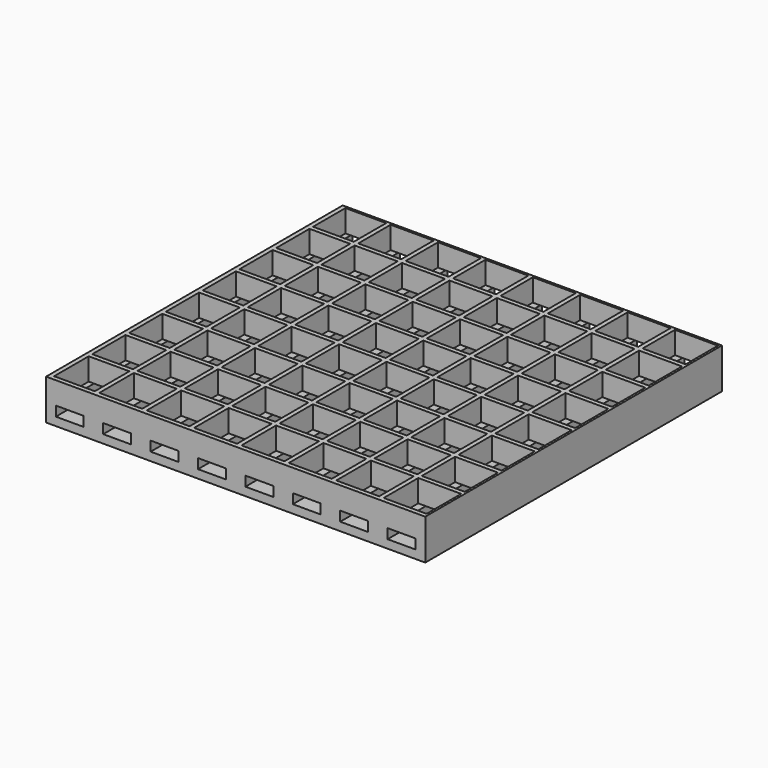
from build123d import *

# Parameters (mm, degrees)
F0_W                 = 3.5
F0_H                 = 3.5
F0_W_2               = 7
F1_DEPTH             = 133
F2_W                 = 1.6
F2_H                 = 8
F2_W_2               = 0.8
F3_DEPTH             = 133
F4_W                 = 0.8
F4_H                 = 8
F4_W_2               = 1.6
F5_DEPTH             = 136
F8_D                 = 3.5
F8_DEPTH             = 12
F8_CSINK_D           = 6.5
F8_CSINK_ANGLE       = 90
F8_TIP               = 1.0515060833
F8_ON_F6_D           = 3.5
F8_ON_F6_DEPTH       = 12
F8_ON_F6_CSINK_D     = 6.5
F8_ON_F6_CSINK_ANGLE = 90
F8_ON_F6_TIP         = 1.0515060833


# Not quite as in the source:
# - a feature names something its author has since deleted; it is built from what else it names


with BuildPart() as f1:
    # F0 (on Front) → F1 (new body)
    with BuildSketch(Plane.XZ):
        with Locations((-66.25, 4.75)):
            Rectangle(F0_W, F0_H)
        with Locations((-17, 4.75)):
            Rectangle(F0_W_2, F0_H)
        with Locations((66.25, 4.75)):
            Rectangle(F0_W, F0_H)
        Polygon((-64.5, 3), (-68, 3), (-68, 0), (68, 0), (68, 3), (64.5, 3), (54.5, 3), (47.5, 3), (37.5, 3), (30.5, 3), (20.5, 3), (13.5, 3), (3.5, 3), (-3.5, 3), (-13.5, 3), (-20.5, 3), (-30.5, 3), (-37.5, 3), (-47.5, 3), (-54.5, 3), align=None)
        with Locations((-51, 4.75)):
            Rectangle(F0_W_2, F0_H)
        with Locations((-34, 4.75)):
            Rectangle(F0_W_2, F0_H)
        with Locations((0, 4.75)):
            Rectangle(F0_W_2, F0_H)
        with Locations((17, 4.75)):
            Rectangle(F0_W_2, F0_H)
        with Locations((34, 4.75)):
            Rectangle(F0_W_2, F0_H)
        with Locations((51, 4.75)):
            Rectangle(F0_W_2, F0_H)
    extrude(amount=F1_DEPTH)

    # F2 (on face) → F3 (join, through all)
    with BuildSketch(Plane.XZ.offset(133)):
        with Locations((-67.2, 10.5)):
            Rectangle(F2_W, F2_H)
        with Locations((-51, 10.5)):
            Rectangle(F2_W, F2_H)
        with Locations((-34, 10.5)):
            Rectangle(F2_W, F2_H)
        with Locations((-17, 10.5)):
            Rectangle(F2_W, F2_H)
        with Locations((0, 10.5)):
            Rectangle(F2_W, F2_H)
        with Locations((17, 10.5)):
            Rectangle(F2_W, F2_H)
        with Locations((34, 10.5)):
            Rectangle(F2_W, F2_H)
        with Locations((51, 10.5)):
            Rectangle(F2_W, F2_H)
        with Locations((67.6, 10.5)):
            Rectangle(F2_W_2, F2_H)
    extrude(amount=-F3_DEPTH)

    # F4 (on face) → F5 (join, through all)
    with BuildSketch(Plane(origin=(-68, 0, 0), x_dir=(0, -1, 0), z_dir=(-1, 0, 0))):
        with Locations((0.4, 10.5)):
            Rectangle(F4_W, F4_H)
        with Locations((16.1, 10.5)):
            Rectangle(F4_W_2, F4_H)
        with Locations((32.6, 10.5)):
            Rectangle(F4_W_2, F4_H)
        with Locations((49.1, 10.5)):
            Rectangle(F4_W_2, F4_H)
        with Locations((65.6, 10.5)):
            Rectangle(F4_W_2, F4_H)
        with Locations((82.1, 10.5)):
            Rectangle(F4_W_2, F4_H)
        with Locations((98.6, 10.5)):
            Rectangle(F4_W_2, F4_H)
        with Locations((115.1, 10.5)):
            Rectangle(F4_W_2, F4_H)
        with Locations((132.2, 10.5)):
            Rectangle(F4_W_2, F4_H)
    extrude(amount=-F5_DEPTH)

    # F8
    with Locations(Plane.XY.offset(3)):
        with Locations((42.5, -42), (42.5, -91)):
            CounterSinkHole(F8_D / 2, F8_CSINK_D / 2, depth=F8_DEPTH, counter_sink_angle=F8_CSINK_ANGLE)
            with Locations((0, 0, -(F8_DEPTH + F8_TIP / 2))):  # 118° drill point
                Cone(0, F8_D / 2, F8_TIP, mode=Mode.SUBTRACT)

    # F8 on F6
    with Locations(Plane.XY.offset(3)):
        with Locations((-42.5, -42), (-42.5, -91)):
            CounterSinkHole(F8_ON_F6_D / 2, F8_ON_F6_CSINK_D / 2, depth=F8_ON_F6_DEPTH, counter_sink_angle=F8_ON_F6_CSINK_ANGLE)
            with Locations((0, 0, -(F8_ON_F6_DEPTH + F8_ON_F6_TIP / 2))):  # 118° drill point
                Cone(0, F8_ON_F6_D / 2, F8_ON_F6_TIP, mode=Mode.SUBTRACT)


solid = f1.part
